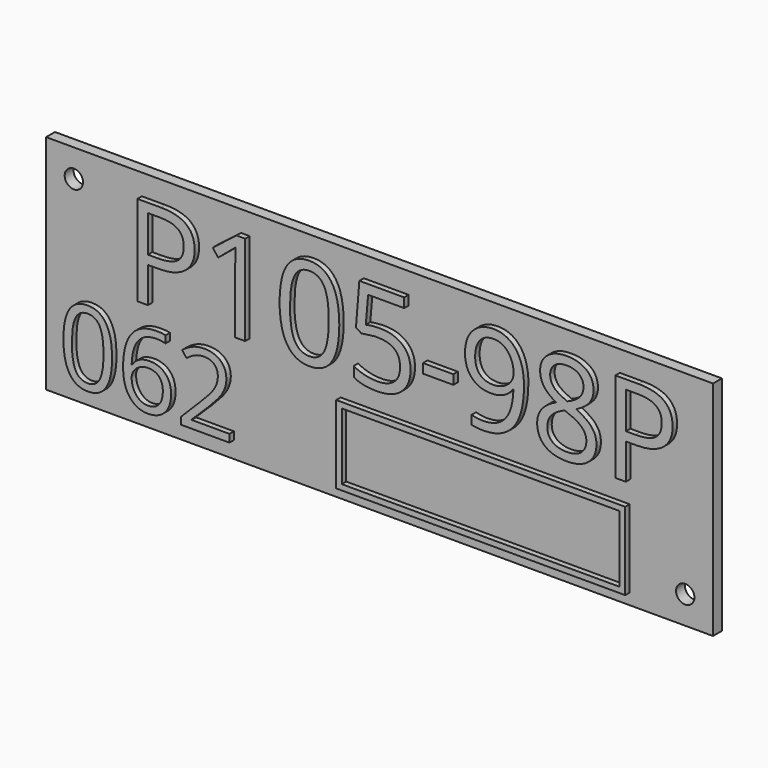
from build123d import *

# Parameters (mm, degrees)
F0_W         = 120
F0_H         = 40
F1_DEPTH     = 2
F3_D         = 3.3
F4_TEXT_SIZE = 22.7377695669
F5_DEPTH     = 1
F6_TEXT_SIZE = 18.5356140827
F7_DEPTH     = 1
F8_W         = 52
F8_H         = 14
F8_W_2       = 49.99999962
F8_H_2       = 11.99999962
F9_DEPTH     = 1


# Not quite as in the source:
# - Text() gives the source's letters only with a copy of the font that has no kerning and outlines rounded to 1/6400 em; it was checked with that copy


with BuildPart() as f1:
    # F0 (on Front) → F1 (new body)
    with BuildSketch(Plane.XZ):
        Rectangle(F0_W, F0_H)
    extrude(amount=F1_DEPTH)

    # F3 (through all)
    with Locations(Plane.XZ.offset(2)):
        with Locations((-55, 15), (55, -15)):
            Hole(F3_D / 2)

    # F4 (on face) → F5 (join)
    with BuildSketch(Plane.XZ.offset(2)):
        with Locations((-45, 0)):
            Text('P105-98P', F4_TEXT_SIZE, font='Open Sans', text_align=(TextAlign.LEFT, TextAlign.BOTTOM))
    extrude(amount=F5_DEPTH)

    # F6 (on face) → F7 (join)
    with BuildSketch(Plane.XZ.offset(2)):
        with Locations((-57, -17)):
            Text('062', F6_TEXT_SIZE, font='Open Sans', text_align=(TextAlign.LEFT, TextAlign.BOTTOM))
    extrude(amount=F7_DEPTH)

    # F8 (on face) → F9 (join)
    with BuildSketch(Plane.XZ.offset(2)):
        with Locations((19, -11)):
            Rectangle(F8_W, F8_H)
        with Locations((19, -11)):
            Rectangle(F8_W_2, F8_H_2, mode=Mode.SUBTRACT)
    extrude(amount=F9_DEPTH)


solid = f1.part
